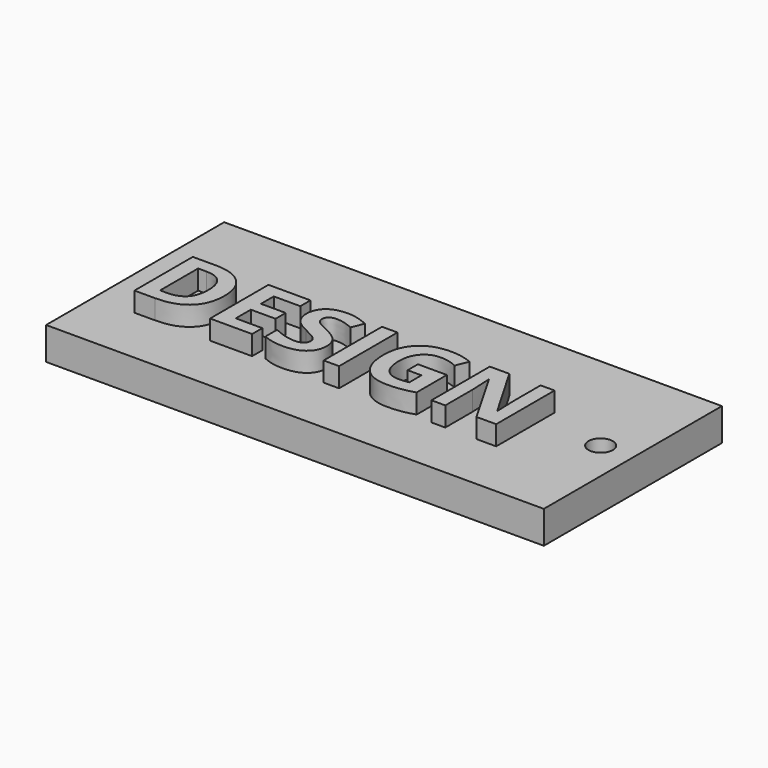
from build123d import *

# Parameters (mm, degrees)
F0_W         = 153.0243456364
F0_H         = 68.4415623546
F0_R         = 3.7401420453
F1_DEPTH     = 10
F2_TEXT_SIZE = 31.4198744794
F3_DEPTH     = 6


# Not quite as in the source:
# - Text() gives the source's letters only with a copy of the font that has no kerning and outlines rounded to 1/6400 em; it was checked with that copy


with BuildPart() as f1:
    # F0 (on Top) → F1 (new body)
    with BuildSketch(Plane.XY):
        with Locations((-43.4603095055, 15.9958638251)):
            Rectangle(F0_W, F0_H)
        with Locations((23.1477469206, 15.9958638251)):
            Circle(F0_R, mode=Mode.SUBTRACT)
    extrude(amount=F1_DEPTH)

    # F2 (on face) → F3 (join)
    with BuildSketch(Plane.XY.offset(10)):
        with Locations((-110.2146189296, 0)):
            Text('DESIGN', F2_TEXT_SIZE, font='Open Sans', font_style=FontStyle.BOLD, text_align=(TextAlign.LEFT, TextAlign.BOTTOM))
    extrude(amount=F3_DEPTH)


solid = f1.part
